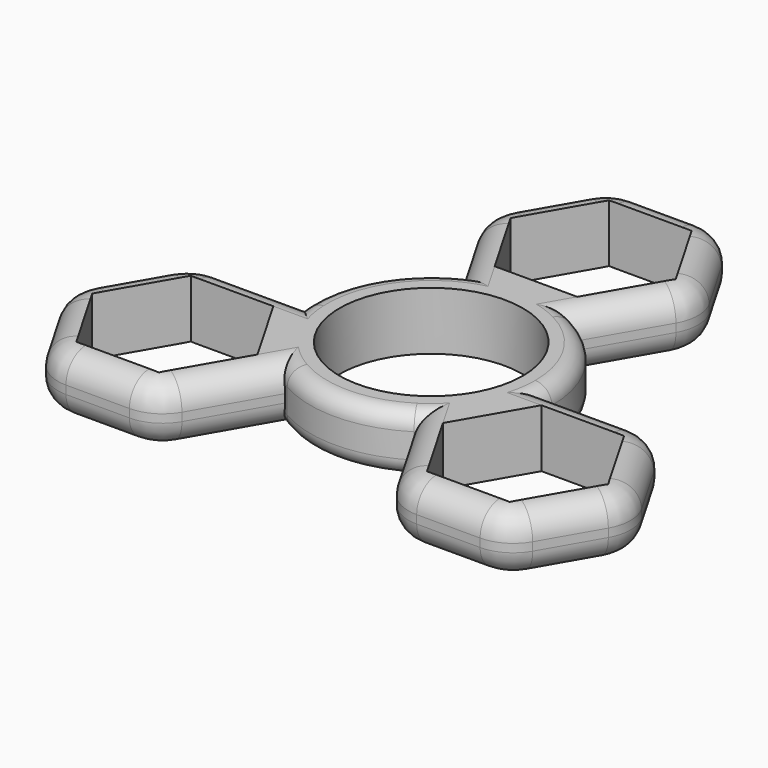
from build123d import *

# Parameters (mm, degrees)
F0_R         = 11.05
F1_DEPTH     = 7
F2_R         = 5
F3_T1_DEPTH  = 17.9282658604
F3_T3_DEPTH  = 7.6498910668
F3_T5_DEPTH  = 7.6498910668
F3_T7_DEPTH  = 17.9282658604
F3_T9_DEPTH  = 7.6498910668
F3_T12_ANGLE = 60
F3_T14_ANGLE = 60
F3_T16_ANGLE = 60
F3_T18_ANGLE = 60
F3_T20_ANGLE = 60
F3_T22_ANGLE = 60
F3_T24_ANGLE = 60
F3_T26_ANGLE = 60
F4_R         = 2
F5_COUNT     = 3


# Not quite as in the source:
# - a fillet or chamfer that OpenCascade refuses, or shapes differently, is made with other operations: its cross-section is extruded or revolved along the edge and cut away or added
# - a feature names something its author has since deleted; it is built from what else it names


with BuildPart() as f1:
    # F0 (on Top) → F1 (new body)
    with BuildSketch(Plane.XY):
        with BuildLine():
            ThreePointArc((-6.7658851555, 12.8811994031), (-7.5252531847, -12.4528335935), (14.55, 0))
            ThreePointArc((14.55, 0), (12.4528335935, 7.5252531847), (6.7658851555, 12.8811994031))
            Line((6.7658851555, 12.8811994031), (6.7116968793, 12.7873425556))
            Line((6.7116968793, 12.7873425556), (-6.7116968793, 12.7873425556))
            Line((-6.7116968793, 12.7873425556), (-6.7658851555, 12.8811994031))
        make_face()
        Circle(F0_R, mode=Mode.SUBTRACT)
        with BuildLine():
            Line((6.7116968793, 12.7873425556), (6.7658851555, 12.8811994031))
            ThreePointArc((6.7658851555, 12.8811994031), (0, 14.55), (-6.7658851555, 12.8811994031))
            Line((-6.7658851555, 12.8811994031), (-6.7116968793, 12.7873425556))
            Line((-6.7116968793, 12.7873425556), (6.7116968793, 12.7873425556))
        make_face()
        with BuildLine():
            ThreePointArc((-6.7658851555, 12.8811994031), (0, 14.55), (6.7658851555, 12.8811994031))
            Line((6.7658851555, 12.8811994031), (13.4233937587, 24.4123425556))
            Line((13.4233937587, 24.4123425556), (6.7116968793, 36.0373425556))
            Line((6.7116968793, 36.0373425556), (-6.7116968793, 36.0373425556))
            Line((-6.7116968793, 36.0373425556), (-13.4233937587, 24.4123425556))
            Line((-13.4233937587, 24.4123425556), (-6.7658851555, 12.8811994031))
        make_face()
        Polygon((-9.9592921435, 24.4123425556), (-4.9796460718, 33.0373425556), (4.9796460718, 33.0373425556), (9.9592921435, 24.4123425556), (4.9796460718, 15.7873425556), (-4.9796460718, 15.7873425556), align=None, mode=Mode.SUBTRACT)
    extrude(amount=F1_DEPTH)

    # F2
    f2_edges = [f1.edges().sort_by_distance(p)[0] for p in [
        (13.423394, 24.412343, 3.5),
        (6.711697, 36.037343, 3.5),
        (-6.711697, 36.037343, 3.5),
        (-13.423394, 24.412343, 3.5),
    ]]
    fillet(f2_edges, radius=F2_R)

    # F3: fillet of radius 3 on 18 edges, made by hand

    # F3_s2 → F3_t1 (cut)
    with BuildSketch(Plane(origin=(3.519194246, 6.0954232358, 0), x_dir=(0, 0, 1), z_dir=(0.5, 0.8660254038, 0))):
        with BuildLine():
            ThreePointArc((3, -0.5811712778), (0.8786796564, -1.4598509343), (0, -3.5811712778))
            Line((0, -3.5811712778), (0, -0.5811712778))
            Line((0, -0.5811712778), (3, -0.5811712778))
        make_face()
        with BuildLine():
            ThreePointArc((4, -0.5811712778), (6.1213203436, -1.4598509343), (7, -3.5811712778))
            Line((7, -3.5811712778), (7, -0.5811712778))
            Line((7, -0.5811712778), (4, -0.5811712778))
        make_face()
    extrude(amount=F3_T1_DEPTH, mode=Mode.SUBTRACT)

    # F3_s4 → F3_t3 (cut)
    with BuildSketch(Plane(origin=(12.4833271762, 21.6217569167, 0), x_dir=(0, 0, 1), z_dir=(-0.5, -0.8660254038, 0))):
        with BuildLine():
            ThreePointArc((7, 20.8311712778), (6.1213203436, 22.9524916214), (4, 23.8311712778))
            Line((4, 23.8311712778), (7, 23.8311712778))
            Line((7, 23.8311712778), (7, 20.8311712778))
        make_face()
        with BuildLine():
            ThreePointArc((0, 20.8311712778), (0.8786796564, 22.9524916214), (3, 23.8311712778))
            Line((3, 23.8311712778), (0, 23.8311712778))
            Line((0, 23.8311712778), (0, 20.8311712778))
        make_face()
    extrude(amount=F3_T3_DEPTH, mode=Mode.SUBTRACT)

    # F3_s6 → F3_t5 (cut)
    with BuildSketch(Plane(origin=(-8.6583816428, 14.9967569167, 0), x_dir=(0, 0, 1), z_dir=(-0.5, 0.8660254038, 0))):
        with BuildLine():
            ThreePointArc((0, 20.8311712778), (0.8786796564, 22.9524916214), (3, 23.8311712778))
            Line((3, 23.8311712778), (0, 23.8311712778))
            Line((0, 23.8311712778), (0, 20.8311712778))
        make_face()
        with BuildLine():
            ThreePointArc((7, 20.8311712778), (6.1213203436, 22.9524916214), (4, 23.8311712778))
            Line((4, 23.8311712778), (7, 23.8311712778))
            Line((7, 23.8311712778), (7, 20.8311712778))
        make_face()
    extrude(amount=F3_T5_DEPTH, mode=Mode.SUBTRACT)

    # F3_s8 → F3_t7 (cut)
    with BuildSketch(Plane(origin=(-12.4833271762, 21.6217569167, 0), x_dir=(0, 0, 1), z_dir=(0.5, -0.8660254038, 0))):
        with BuildLine():
            ThreePointArc((0, -3.5811712778), (0.8786796564, -1.4598509343), (3, -0.5811712778))
            Line((3, -0.5811712778), (0, -0.5811712778))
            Line((0, -0.5811712778), (0, -3.5811712778))
        make_face()
        with BuildLine():
            ThreePointArc((7, -3.5811712778), (6.1213203436, -1.4598509343), (4, -0.5811712778))
            Line((4, -0.5811712778), (7, -0.5811712778))
            Line((7, -0.5811712778), (7, -3.5811712778))
        make_face()
    extrude(amount=F3_T7_DEPTH, mode=Mode.SUBTRACT)

    # F3_s10 → F3_t9 (cut)
    with BuildSketch(Plane.YZ.offset(-3.8249455334)):
        with BuildLine():
            ThreePointArc((33.0373425556, 0), (35.1586628992, 0.8786796564), (36.0373425556, 3))
            Line((36.0373425556, 3), (36.0373425556, 0))
            Line((36.0373425556, 0), (33.0373425556, 0))
        make_face()
        with BuildLine():
            ThreePointArc((33.0373425556, 7), (35.1586628992, 6.1213203436), (36.0373425556, 4))
            Line((36.0373425556, 4), (36.0373425556, 7))
            Line((36.0373425556, 7), (33.0373425556, 7))
        make_face()
    extrude(amount=F3_T9_DEPTH, mode=Mode.SUBTRACT)

    # F3_s11 → F3_t12 (revolve, cut)
    with BuildSketch(Plane(origin=(12.4833271762, 21.6217569167, 0), x_dir=(0, 0, 1), z_dir=(-0.5, -0.8660254038, 0))):
        with BuildLine():
            ThreePointArc((0, 3.5811712778), (0.8786796564, 1.4598509343), (3, 0.5811712778))
            Line((3, 0.5811712778), (0, 0.5811712778))
            Line((0, 0.5811712778), (0, 3.5811712778))
        make_face()
    revolve(axis=Axis((7.6498910668, 24.4123425556, 0), (0, 0, 1)), revolution_arc=F3_T12_ANGLE, mode=Mode.SUBTRACT)

    # F3_s13 → F3_t14 (revolve, cut)
    with BuildSketch(Plane(origin=(-12.4833271762, 21.6217569167, 0), x_dir=(0, 0, 1), z_dir=(0.5, -0.8660254038, 0))):
        with BuildLine():
            ThreePointArc((0, -20.8311712778), (0.8786796564, -22.9524916214), (3, -23.8311712778))
            Line((3, -23.8311712778), (0, -23.8311712778))
            Line((0, -23.8311712778), (0, -20.8311712778))
        make_face()
    revolve(axis=Axis((3.8249455334, 31.0373425556, 0), (0, 0, 1)), revolution_arc=F3_T14_ANGLE, mode=Mode.SUBTRACT)

    # F3_s15 → F3_t16 (revolve, cut)
    with BuildSketch(Plane(origin=(8.6583816428, 14.9967569167, 0), x_dir=(0, 0, 1), z_dir=(0.5, 0.8660254038, 0))):
        with BuildLine():
            ThreePointArc((0, -20.8311712778), (0.8786796564, -22.9524916214), (3, -23.8311712778))
            Line((3, -23.8311712778), (0, -23.8311712778))
            Line((0, -23.8311712778), (0, -20.8311712778))
        make_face()
    revolve(axis=Axis((-7.6498910668, 24.4123425556, 0), (0, 0, 1)), revolution_arc=F3_T16_ANGLE, mode=Mode.SUBTRACT)

    # F3_s17 → F3_t18 (revolve, cut)
    with BuildSketch(Plane.YZ.offset(-3.8249455334)):
        with BuildLine():
            ThreePointArc((33.0373425556, 0), (35.1586628992, 0.8786796564), (36.0373425556, 3))
            Line((36.0373425556, 3), (36.0373425556, 0))
            Line((36.0373425556, 0), (33.0373425556, 0))
        make_face()
    revolve(axis=Axis((-3.8249455334, 31.0373425556, 0), (0, 0, 1)), revolution_arc=F3_T18_ANGLE, mode=Mode.SUBTRACT)

    # F3_s19 → F3_t20 (revolve, cut)
    with BuildSketch(Plane(origin=(12.4833271762, 21.6217569167, 0), x_dir=(0, 0, 1), z_dir=(-0.5, -0.8660254038, 0))):
        with BuildLine():
            ThreePointArc((4, 0.5811712778), (6.1213203436, 1.4598509343), (7, 3.5811712778))
            Line((7, 3.5811712778), (7, 0.5811712778))
            Line((7, 0.5811712778), (4, 0.5811712778))
        make_face()
    revolve(axis=Axis((7.6498910668, 24.4123425556, 7), (0, 0, 1)), revolution_arc=F3_T20_ANGLE, mode=Mode.SUBTRACT)

    # F3_s21 → F3_t22 (revolve, cut)
    with BuildSketch(Plane(origin=(-12.4833271762, 21.6217569167, 0), x_dir=(0, 0, 1), z_dir=(0.5, -0.8660254038, 0))):
        with BuildLine():
            ThreePointArc((7, -20.8311712778), (6.1213203436, -22.9524916214), (4, -23.8311712778))
            Line((4, -23.8311712778), (7, -23.8311712778))
            Line((7, -23.8311712778), (7, -20.8311712778))
        make_face()
    revolve(axis=Axis((3.8249455334, 31.0373425556, 7), (0, 0, 1)), revolution_arc=F3_T22_ANGLE, mode=Mode.SUBTRACT)

    # F3_s23 → F3_t24 (revolve, cut)
    with BuildSketch(Plane(origin=(8.6583816428, 14.9967569167, 0), x_dir=(0, 0, 1), z_dir=(0.5, 0.8660254038, 0))):
        with BuildLine():
            ThreePointArc((7, -20.8311712778), (6.1213203436, -22.9524916214), (4, -23.8311712778))
            Line((4, -23.8311712778), (7, -23.8311712778))
            Line((7, -23.8311712778), (7, -20.8311712778))
        make_face()
    revolve(axis=Axis((-7.6498910668, 24.4123425556, 7), (0, 0, 1)), revolution_arc=F3_T24_ANGLE, mode=Mode.SUBTRACT)

    # F3_s25 → F3_t26 (revolve, cut)
    with BuildSketch(Plane.YZ.offset(-3.8249455334)):
        with BuildLine():
            ThreePointArc((33.0373425556, 7), (35.1586628992, 6.1213203436), (36.0373425556, 4))
            Line((36.0373425556, 4), (36.0373425556, 7))
            Line((36.0373425556, 7), (33.0373425556, 7))
        make_face()
    revolve(axis=Axis((-3.8249455334, 31.0373425556, 7), (0, 0, 1)), revolution_arc=F3_T26_ANGLE, mode=Mode.SUBTRACT)

    # F4
    f4_edges = [f1.edges().sort_by_distance(p)[0] for p in [
        (0, -14.55, 7),
        (0, -14.55, 0),
    ]]
    fillet(f4_edges, radius=F4_R)

    # F5: F1 ×3 about axis
    f5_axis = Axis((0, 0, 0), (0, 0, -1))


with BuildPart() as f1_1:
    add(f1.part)
    for i in range(1, F5_COUNT):
        add(f1.part.rotate(f5_axis, i * 360 / F5_COUNT))


solid = f1_1.part
